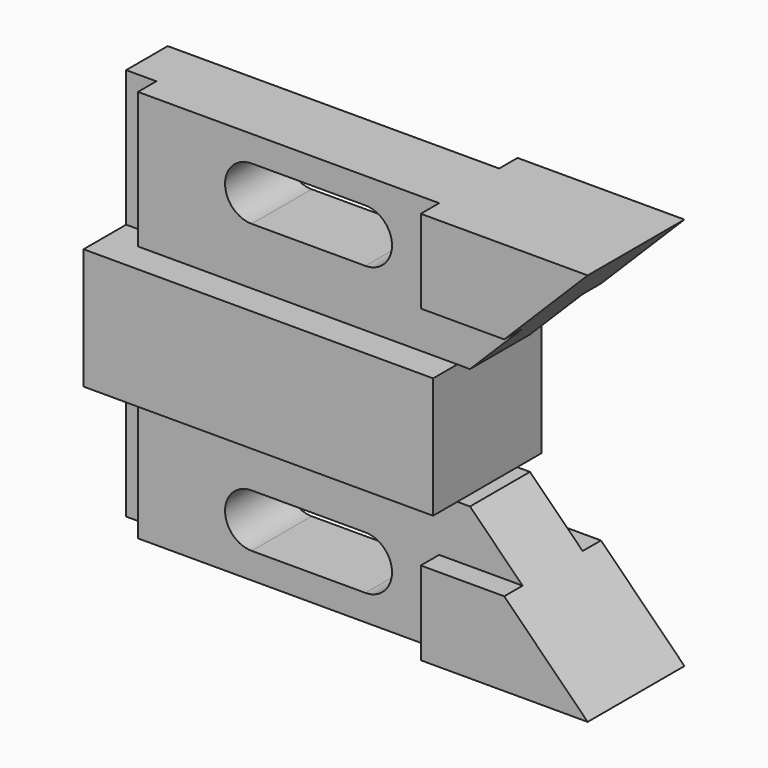
from build123d import *

# Parameters (mm, degrees)
F0_W     = 73.406
F0_H     = 25.4
F1_DEPTH = 14.224
F2_W     = 31.242
F2_H     = 25.4
F3_DEPTH = 28.575
F5_DEPTH = 22.099
F6_W     = 4.826
F6_H     = 11.049
F7_DEPTH = 104.649
F9_DEPTH = 26.925


# Not quite as in the source:
# - a pattern or mirror of a feature is missing from the dataset's text; its kind, count and spacing are read off the source's solid


with BuildPart() as f1:
    # F0 (on Front) → F1 (new body, symmetric)
    with BuildSketch(Plane.XZ):
        Rectangle(F0_W, F0_H)
    extrude(amount=F1_DEPTH, both=True)

    # F2 (on face) → F3 (join)
    with BuildSketch(Plane.XY.offset(12.7)):
        Polygon((-36.703, 7.874), (-36.703, -3.048), (-30.353, -3.048), (-30.353, -7.874), (32.893, -7.874), (32.893, -12.7), (36.703, -12.7), (36.703, 12.7), (32.893, 12.7), (32.893, 7.874), align=None)
        with Locations((52.324, 0)):
            Rectangle(F2_W, F2_H)
    f3 = extrude(amount=F3_DEPTH)

    # F3_copies: F3 across plane
    add(f3.mirror(Plane(origin=(0, 0, 0), x_dir=(-1, 0, 0), z_dir=(0, 0, -1))))

    # F4 (on face) → F5 (cut, through all)
    with BuildSketch(Plane.XZ.offset(7.874)):
        with BuildLine():
            ThreePointArc((-6.477, 35.814), (-12.065, 30.226), (-6.477, 24.638))
            Line((-6.477, 24.638), (17.399, 24.638))
            ThreePointArc((17.399, 24.638), (22.987, 30.226), (17.399, 35.814))
            Line((17.399, 35.814), (-6.477, 35.814))
        make_face()
    f5 = extrude(amount=-F5_DEPTH, mode=Mode.SUBTRACT)

    # F5_copies: F5 across plane
    add(f5.mirror(Plane(origin=(0, 0, 0), x_dir=(-1, 0, 0), z_dir=(0, 0, -1))), mode=Mode.SUBTRACT)

    # F6 (on face) → F7 (cut, through all)
    with BuildSketch(Plane.YZ.offset(67.945)):
        with Locations((-10.287, 18.2245)):
            Rectangle(F6_W, F6_H)
        with Locations((10.287, 18.2245)):
            Rectangle(F6_W, F6_H)
    f7 = extrude(amount=-F7_DEPTH, mode=Mode.SUBTRACT)

    # F7_copies: F7 across plane
    add(f7.mirror(Plane(origin=(0, 0, 0), x_dir=(-1, 0, 0), z_dir=(0, 0, -1))), mode=Mode.SUBTRACT)

    # F8 (on face) → F9 (cut, through all)
    with BuildSketch(Plane.XZ.offset(12.7)):
        Polygon((67.945, 41.275), (50.419, 23.749), (67.945, 23.749), align=None)
        Polygon((50.419, 23.749), (39.37, 12.7), (67.945, 12.7), (67.945, 23.749), align=None)
    f9 = extrude(amount=-F9_DEPTH, mode=Mode.SUBTRACT)

    # F9_copies: F9 across plane
    add(f9.mirror(Plane(origin=(0, 0, 0), x_dir=(-1, 0, 0), z_dir=(0, 0, -1))), mode=Mode.SUBTRACT)


solid = f1.part
